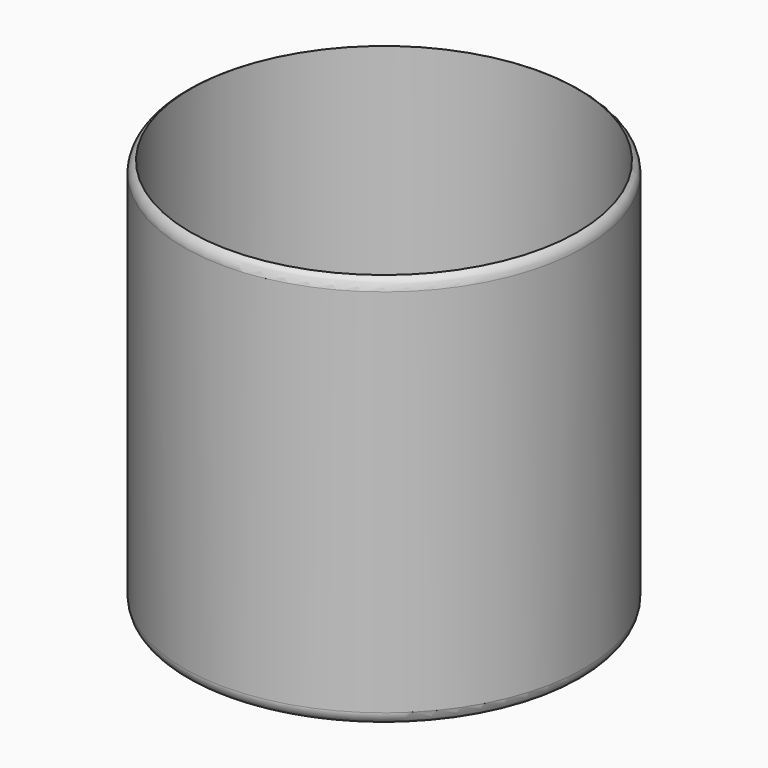
from build123d import *

# Parameters (mm, degrees)
F0_R     = 77.2459494585
F1_DEPTH = 152.4
F2_T     = -2.54


# Not quite as in the source:
# - a fillet or chamfer that OpenCascade refuses, or shapes differently, is made with other operations: its cross-section is extruded or revolved along the edge and cut away or added


with BuildPart() as f1:
    # F0 (on Top) → F1 (new body)
    with BuildSketch(Plane.XY):
        Circle(F0_R)
    extrude(amount=F1_DEPTH)

    # F2
    f2_openings = [f1.faces().sort_by_distance(p)[0] for p in [
        (0, 0, 152.4),
    ]]
    offset(amount=F2_T, openings=f2_openings)

    # F3: fillet of radius 5.08 on 3 edges, made by hand

    # F3_s1 → F3_t2 (revolve, cut)
    with BuildSketch(Plane.XZ):
        with BuildLine():
            ThreePointArc((77.2459494585, 5.08), (75.758051907, 1.4878975516), (72.1659494585, 0))
            Line((72.1659494585, 0), (72.1659494585, -0.1016))
            Line((72.1659494585, -0.1016), (77.3475494585, -0.1016))
            Line((77.3475494585, -0.1016), (77.3475494585, 5.08))
            Line((77.3475494585, 5.08), (77.2459494585, 5.08))
        make_face()
    revolve(axis=Axis((0, 0, 0), (0, 0, 1)), mode=Mode.SUBTRACT)

    # F3_s3 → F3_t4 (revolve, cut)
    with BuildSketch(Plane.XZ):
        with BuildLine():
            ThreePointArc((77.2459494585, 148.0005909488), (76.5653585098, 150.5405909488), (74.7059494585, 152.4))
            Line((74.7059494585, 152.4), (74.7567494585, 152.487988181))
            ThreePointArc((74.7567494585, 152.487988181), (75.9759494585, 152.5016), (77.2459494585, 152.5016))
            Line((77.2459494585, 152.5016), (77.3475494585, 152.4))
            Line((77.3475494585, 152.4), (77.3475494585, 148.0005909488))
            Line((77.3475494585, 148.0005909488), (77.2459494585, 148.0005909488))
        make_face()
    revolve(axis=Axis((0, 0, 152.4), (0, 0, 1)), mode=Mode.SUBTRACT)


solid = f1.part
